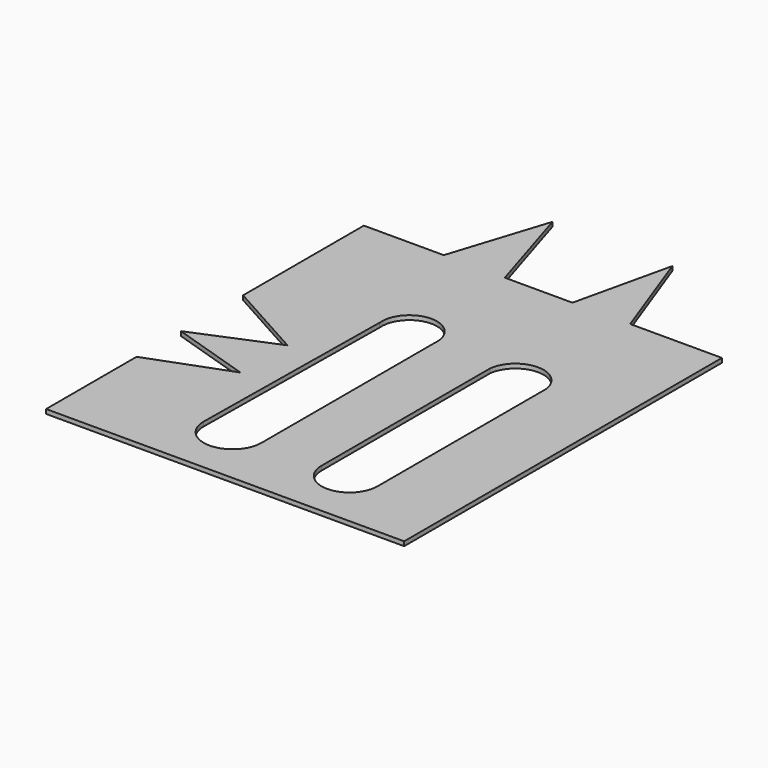
from build123d import *

# Parameters (mm, degrees)
F1_DEPTH = 1


# Not quite as in the source:
# - ends of sketch curves that miss each other by under 0.0002 mm in the source are joined


with BuildPart() as f1:
    # F0 (on Top) → F1 (new body)
    with BuildSketch(Plane.XY):
        Polygon((28.8763996214, 52.6419393718), (20.6990148872, 75), (15.5881475657, 52.6419393718), (0, 52.6419393718), (-6.8996730261, 75), (-14.0548860654, 52.6419393718), (-32.458178699, 52.6419393718), (-32.458178699, 17.8880356252), (-14.0548860654, 7.6663014479), (-32.458178699, 0), (-14.0548860654, -5.889575201), (-32.458178699, -12.7771692351), (-32.458178699, -38.8200990856), (50, -38.8200990856), (50, 52.6419393718), align=None)
        with BuildLine():
            ThreePointArc((-6.6301580518, 24.9263830483), (-0.2351544327, 31.911792251), (6.0177850537, 24.7989334166))
            Line((6.0177850537, 24.7989334166), (6.0177850537, -24.9158367515))
            ThreePointArc((6.0177850537, -24.9158367515), (-0.631557079, -31.5651788842), (-7.2808992118, -24.9158367515))
            Line((-7.2808992118, -24.9158367515), (-6.6301580518, 24.9263830483))
        make_face(mode=Mode.SUBTRACT)
        with BuildLine():
            ThreePointArc((20.0069602579, 23.4479047358), (26.4433873817, 29.1369264448), (32.8798145056, 23.4479047358))
            Line((32.8798145056, 23.4479047358), (32.8798145056, -25.096591562))
            ThreePointArc((32.8798145056, -25.096591562), (26.443391107, -31.5330224112), (20.0069602579, -25.096591562))
            Line((20.0069602579, -25.096591562), (20.0069602579, 23.4479047358))
        make_face(mode=Mode.SUBTRACT)
    extrude(amount=F1_DEPTH)


solid = f1.part
